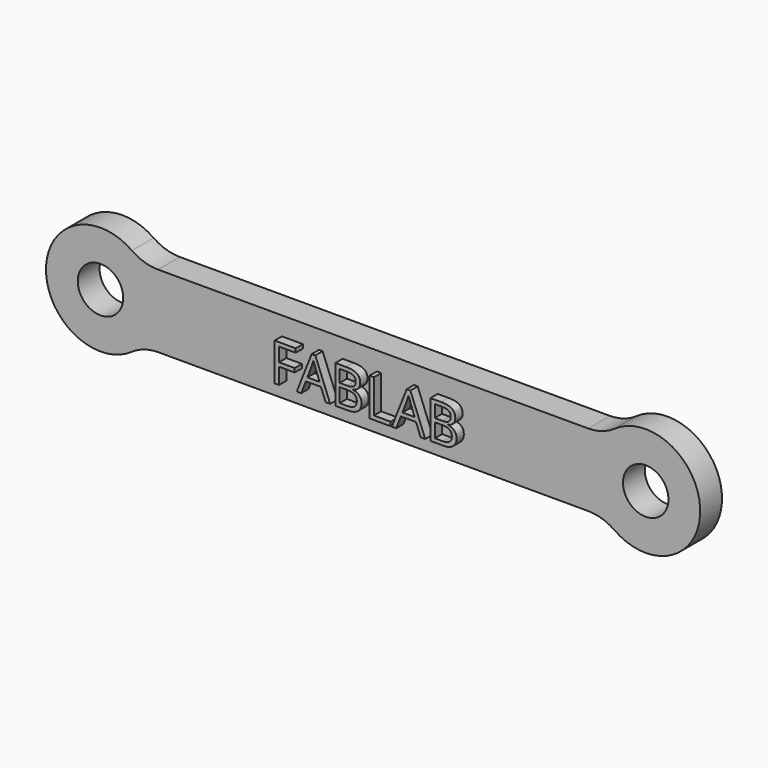
from build123d import *

# Parameters (mm, degrees)
F0_R         = 2.5
F1_DEPTH     = 3
F2_TEXT_SIZE = 5.8114842331
F3_DEPTH     = 1


# Not quite as in the source:
# - Text() gives the source's letters only with a copy of the font that has no kerning and outlines rounded to 1/6400 em; it was checked with that copy


with BuildPart() as f1:
    # F0 (on Front) → F1 (new body)
    with BuildSketch(Plane.XZ):
        with BuildLine():
            ThreePointArc((6.3245553203, 4), (4.8169985974, 4.2326870538), (3.4497574475, 4.9090909091))
            ThreePointArc((3.4497574475, 4.9090909091), (-6, 0), (3.4497574475, -4.9090909091))
            ThreePointArc((3.4497574475, -4.9090909091), (4.8169985974, -4.2326870538), (6.3245553203, -4))
            Line((6.3245553203, -4), (53.6754446797, -4))
            ThreePointArc((53.6754446797, -4), (55.1830014026, -4.2326870538), (56.5502425525, -4.9090909091))
            ThreePointArc((56.5502425525, -4.9090909091), (66, 0), (56.5502425525, 4.9090909091))
            ThreePointArc((56.5502425525, 4.9090909091), (55.1830014026, 4.2326870538), (53.6754446797, 4))
            Line((53.6754446797, 4), (6.3245553203, 4))
        make_face()
        Circle(F0_R, mode=Mode.SUBTRACT)
        with Locations((60, 0)):
            Circle(F0_R, mode=Mode.SUBTRACT)
    extrude(amount=F1_DEPTH)

    # F2 (on face) → F3 (join)
    with BuildSketch(Plane.XZ.offset(3)):
        with Locations((19.3999195471, -2.1857144311)):
            Text('FABLAB', F2_TEXT_SIZE, font='Open Sans', text_align=(TextAlign.LEFT, TextAlign.BOTTOM))
    extrude(amount=F3_DEPTH)


solid = f1.part
